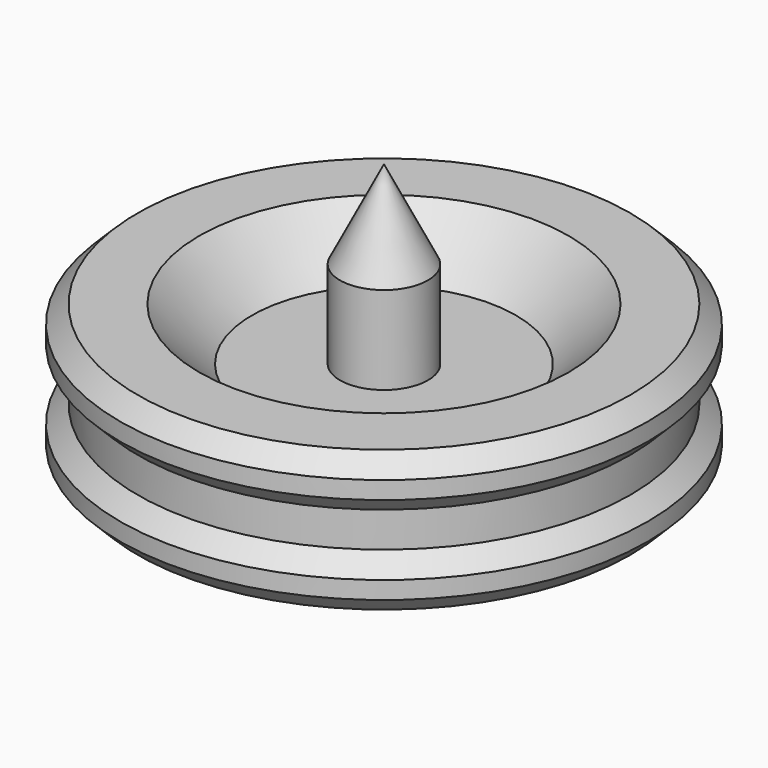
from build123d import *

# Parameters (mm, degrees)
F0_R     = 14
F1_DEPTH = 1
F2_R     = 15
F2_R_2   = 14
F2_R_3   = 7.5
F3_DEPTH = 3
F2_R_4   = 2.5
F4_DEPTH = 10
F5_SIZE  = 0.99999
F6_SIZE  = 2.99999
F7_SIZE2 = 5
F7_SIZE  = 2.5


# Not quite as in the source:
# - a fillet or chamfer is up to 0.001 mm smaller than in the source, because OpenCascade refuses the exact size


with BuildPart() as f1:
    # F0 (on Top) → F1 (new body)
    with BuildSketch(Plane.XY):
        Circle(F0_R)
    extrude(amount=F1_DEPTH)

    # F2 (on face) → F3 (join)
    with BuildSketch(Plane.XY.offset(1)):
        Circle(F2_R)
        Circle(F2_R_2, mode=Mode.SUBTRACT)
        Circle(F2_R_2)
        Circle(F2_R_3, mode=Mode.SUBTRACT)
    extrude(amount=F3_DEPTH)

    # F2 (on face) → F4 (join)
    with BuildSketch(Plane.XY.offset(1)):
        Circle(F2_R_4)
    extrude(amount=F4_DEPTH)

    # F5 (size 1 in the source; OpenCascade refuses exactly that, so slightly less here)
    f5_edges = [f1.edges().sort_by_distance(p)[0] for p in [
        (-15, 0, 4),
        (-15, 0, 1),
    ]]
    chamfer(f5_edges, length=F5_SIZE)

    # F6 (size 3 in the source; OpenCascade refuses exactly that, so slightly less here)
    f6_edges = [f1.edges().sort_by_distance(p)[0] for p in [
        (-7.5, 0, 4),
    ]]
    chamfer(f6_edges, length=F6_SIZE)

    # F7
    f7_edges = [f1.edges().sort_by_distance(p)[0] for p in [
        (-2.5, 0, 11),
    ]]
    f7_side = f1.faces().sort_by_distance((0, 0, 11))[0]
    chamfer(f7_edges, length=F7_SIZE, length2=F7_SIZE2, reference=f7_side)

    # F8: F1 across plane


with BuildPart() as f1_1:
    add(f1.part)
    add(f1.part.mirror(Plane.XY))


solid = f1_1.part
